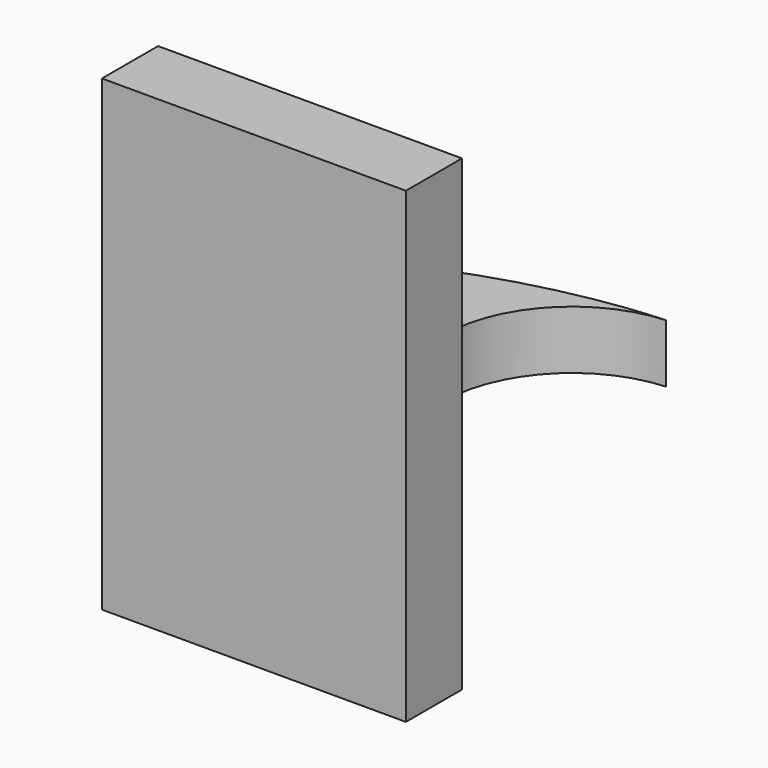
from build123d import *

# Parameters (mm, degrees)
F1_DEPTH = 63.5
F0_W     = 25.4
F0_H     = 28.575
F2_DEPTH = 25.4
F3_DEPTH = 7.9375


# Not quite as in the source:
# - a feature of the source that left no trace in its solid (it failed there, or was rolled back) is left out


with BuildPart() as f1:
    # F0 (on Top) → F1 (new body, symmetric)
    with BuildSketch(Plane.XY):
        Polygon((41.275, -9.525), (41.275, 9.525), (22.225, 9.525), (-41.275, 9.525), (-41.275, -9.525), align=None)
    extrude(amount=F1_DEPTH, both=True)

    # F0 (on Top) → F2 (cut, symmetric)
    with BuildSketch(Plane.XY):
        with BuildLine():
            Line((22.225, 9.525), (41.275, 9.525))
            Line((41.275, 9.525), (41.275, 27.0002))
            ThreePointArc((41.275, 27.0002), (45.9246798487, 38.2255201513), (57.15, 42.8752))
            Line((57.15, 42.8752), (60.325, 42.8752))
            Line((60.325, 42.8752), (60.325, 61.9252))
            Line((60.325, 61.9252), (57.15, 61.9252))
            add(Edge.make_bspline(
                [(54.8307298061, 61.8481068348), (55.6137268289, 61.8824254321), (56.3870657784, 61.908135928), (57.15, 61.9252)],
                knots=[109.0533920202, 109.0533920202, 109.0533920202, 109.0533920202, 111.5045361635, 111.5045361635, 111.5045361635, 111.5045361635], degree=3))
            ThreePointArc((54.8307298061, 61.8481068348), (31.6474889813, 50.8618335723), (22.225, 27.0002))
            Line((22.225, 27.0002), (22.225, 9.525))
        make_face()
        with Locations((98.425, 52.3875)):
            Rectangle(F0_W, F0_H)
        Polygon((60.325, 61.9252), (60.325, 42.8752), (60.325, 38.1), (85.725, 38.1), (85.725, 66.675), (60.325, 66.675), align=None)
    extrude(amount=F2_DEPTH, both=True, mode=Mode.SUBTRACT)


with BuildPart() as f3:
    # F0 (on Top) → F3 (new body, symmetric)
    with BuildSketch(Plane.XY):
        with BuildLine():
            Line((-41.275, 9.525), (22.225, 9.525))
            Line((22.225, 9.525), (22.225, 27.0002))
            ThreePointArc((22.225, 27.0002), (31.6474889813, 50.8618335723), (54.8307298061, 61.8481068348))
            add(Edge.make_bspline(
                [(-41.275, 9.525), (-33.959118263, 41.7552285314), (19.9945568679, 60.3212445943), (54.8307298061, 61.8481068348)],
                knots=[0, 0, 0, 0, 109.0533920202, 109.0533920202, 109.0533920202, 109.0533920202], degree=3))
        make_face()
    extrude(amount=F3_DEPTH, both=True)


solid = Compound([f1.part, f3.part])
